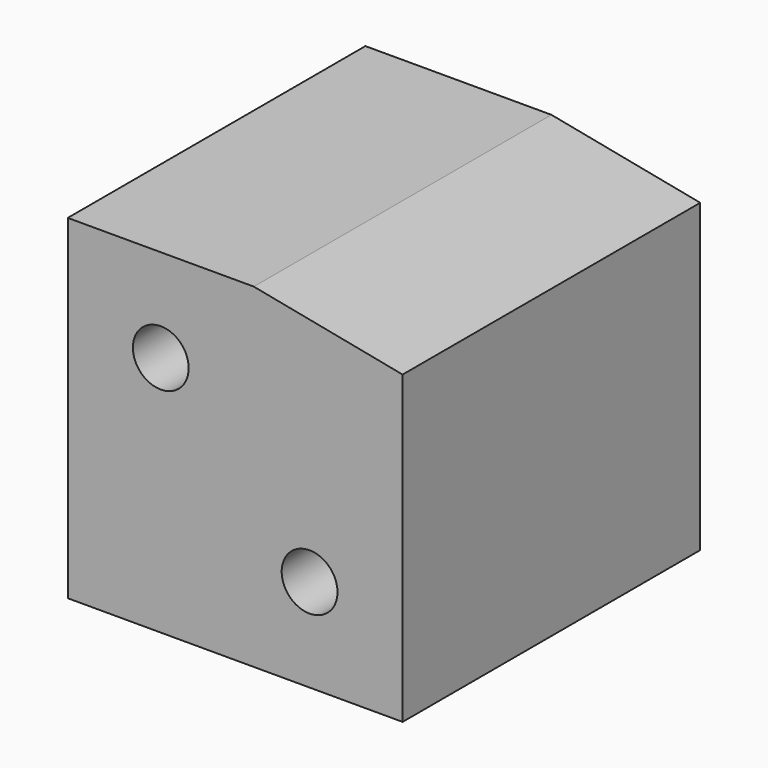
from build123d import *

# Parameters (mm, degrees)
F0_R     = 1.5
F1_DEPTH = 10


# Not quite as in the source:
# - a feature names something its author has since deleted; it is built from what else it names


with BuildPart() as f1:
    # F0 (on Front) → F1 (new body, symmetric)
    with BuildSketch(Plane.XZ):
        Polygon((-5, 24), (-5, 6), (13, 6), (13, 22.4390243902), (5, 24), align=None)
        with Locations((8, 11)):
            Circle(F0_R, mode=Mode.SUBTRACT)
        with Locations((0, 19)):
            Circle(F0_R, mode=Mode.SUBTRACT)
    extrude(amount=F1_DEPTH, both=True)


solid = f1.part
